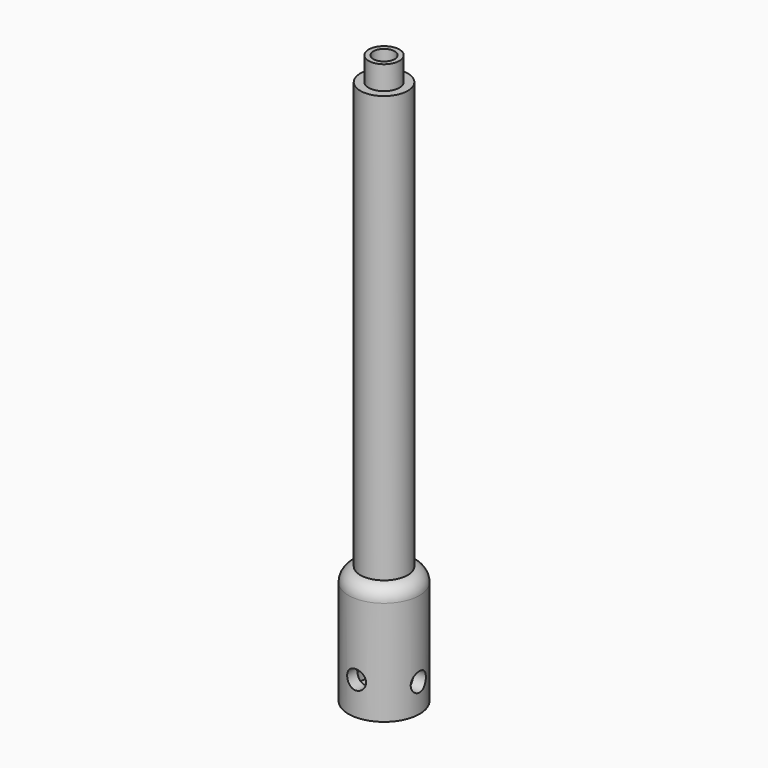
from build123d import *

# Parameters (mm, degrees)
F0_R      = 3.25
F0_R_2    = 2.25
F1_DEPTH  = 100
F0_R_3    = 5
F2_DEPTH  = 95
F0_R_4    = 7.5
F3_DEPTH  = 5
F4_DEPTH  = 20
F6_R      = 5.5
F7_DEPTH  = 2
F8_R      = 2
F9_DEPTH  = 12.5
F10_R     = 2
F11_DEPTH = 12.5


# Not quite as in the source:
# - a fillet or chamfer that OpenCascade refuses, or shapes differently, is made with other operations: its cross-section is extruded or revolved along the edge and cut away or added


with BuildPart() as f1:
    # F0 (on Top) → F1 (new body)
    with BuildSketch(Plane.XY):
        Circle(F0_R)
        Circle(F0_R_2, mode=Mode.SUBTRACT)
    extrude(amount=F1_DEPTH)

    # F0 (on Top) → F2 (join)
    with BuildSketch(Plane.XY):
        Circle(F0_R_3)
        Circle(F0_R, mode=Mode.SUBTRACT)
    extrude(amount=F2_DEPTH)

    # F0 (on Top) → F3 (join)
    with BuildSketch(Plane.XY):
        Circle(F0_R_4)
        Circle(F0_R_3, mode=Mode.SUBTRACT)
    extrude(amount=F3_DEPTH)

    # F0 (on Top) → F4 (join)
    with BuildSketch(Plane.XY):
        Circle(F0_R_4)
        Circle(F0_R_3, mode=Mode.SUBTRACT)
    extrude(amount=-F4_DEPTH)

    # F6 (on offset) → F7 (join)
    with BuildSketch(Plane(origin=(0, 0, -20), x_dir=(1, 0, 0), z_dir=(0, 0, -1))):
        Circle(F6_R)
    extrude(amount=-F7_DEPTH)

    # F8 (on Front) → F9 (cut, symmetric)
    with BuildSketch(Plane.XZ):
        with Locations((0, -13)):
            Circle(F8_R)
    extrude(amount=F9_DEPTH, both=True, mode=Mode.SUBTRACT)

    # F10 (on Right) → F11 (cut, symmetric)
    with BuildSketch(Plane.YZ):
        with Locations((0, -14)):
            Circle(F10_R)
    extrude(amount=F11_DEPTH, both=True, mode=Mode.SUBTRACT)

    # F12: fillet of radius 3 on 1 edges, made by hand

    # F12_s1 → F12_t2 (revolve, cut)
    with BuildSketch(Plane.XZ):
        with BuildLine():
            ThreePointArc((5, 5), (6.7912878475, 3.9784517816), (7.5, 2.0419601084))
            Line((7.5, 2.0419601084), (7.5, 5))
            Line((7.5, 5), (5, 5))
        make_face()
    revolve(axis=Axis((0, 0, 5), (0, 0, 1)), mode=Mode.SUBTRACT)


solid = f1.part
